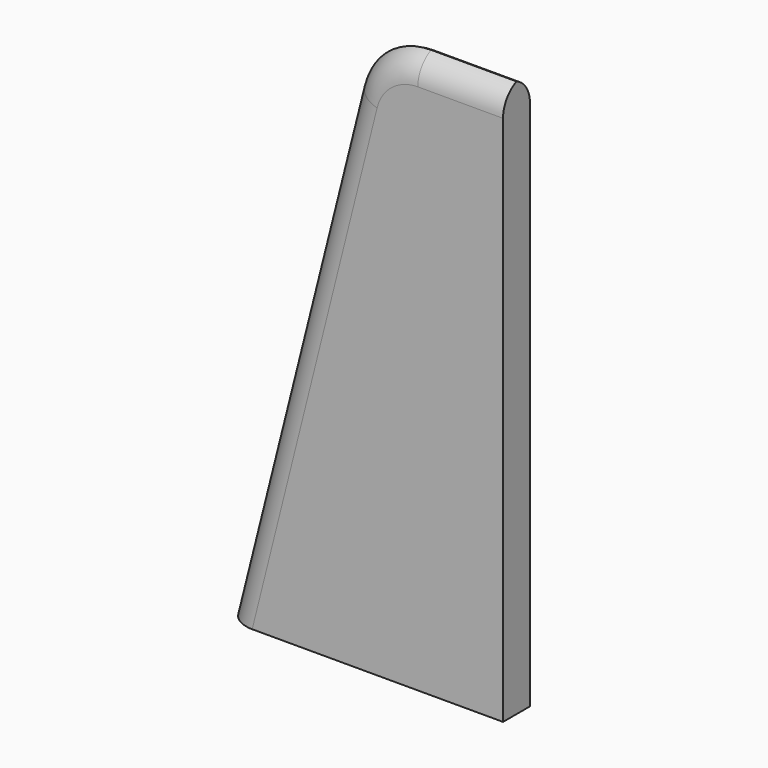
from build123d import *

# Parameters (mm, degrees)
F1_DEPTH    = 3.048
F2_T1_DEPTH = 53.7555112647
F2_T3_DEPTH = 14.0920698193
F2_T6_ANGLE = 75.9637565321
F2_T8_ANGLE = 75.9637565321


# Not quite as in the source:
# - a fillet or chamfer that OpenCascade refuses, or shapes differently, is made with other operations: its cross-section is extruded or revolved along the edge and cut away or added


with BuildPart() as f1:
    # F0 (on Front) → F1 (new body)
    with BuildSketch(Plane.XZ):
        with BuildLine():
            Line((25.4, 50.8), (17.6579301807, 50.8))
            ThreePointArc((17.6579301807, 50.8), (13.750062651, 49.4551045314), (11.4975253047, 45.990101219))
            Line((11.4975253047, 45.990101219), (0, 0))
            Line((0, 0), (25.4, 0))
            Line((25.4, 0), (25.4, 50.8))
        make_face()
    extrude(amount=F1_DEPTH)

    # F2: fillet of radius 2.54 on 2 edges, made by hand

    # F2_s2 → F2_t1 (cut)
    with BuildSketch(Plane(origin=(11.4975253047, 0, 45.990101219), x_dir=(0, 1, 0), z_dir=(-0.242535625, 0, -0.9701425001))):
        with BuildLine():
            ThreePointArc((-0.508, 0), (-2.3040512242, 0.7439487758), (-3.048, 2.54))
            Line((-3.048, 2.54), (-3.048, 0))
            Line((-3.048, 0), (-0.508, 0))
        make_face()
        with BuildLine():
            ThreePointArc((-2.54, 0), (-0.7439487758, 0.7439487758), (0, 2.54))
            Line((0, 2.54), (0, 0))
            Line((0, 0), (-2.54, 0))
        make_face()
    extrude(amount=F2_T1_DEPTH, mode=Mode.SUBTRACT)

    # F2_s4 → F2_t3 (cut)
    with BuildSketch(Plane.YZ.offset(17.6579301807)):
        with BuildLine():
            ThreePointArc((-2.54, 50.8), (-0.7439487758, 50.0560512242), (0, 48.26))
            Line((0, 48.26), (0, 50.8))
            Line((0, 50.8), (-2.54, 50.8))
        make_face()
        with BuildLine():
            ThreePointArc((-0.508, 50.8), (-2.3040512242, 50.0560512242), (-3.048, 48.26))
            Line((-3.048, 48.26), (-3.048, 50.8))
            Line((-3.048, 50.8), (-0.508, 50.8))
        make_face()
    extrude(amount=F2_T3_DEPTH, mode=Mode.SUBTRACT)

    # F2_s5 → F2_t6 (revolve, cut)
    with BuildSketch(Plane.YZ.offset(17.6579301807)):
        with BuildLine():
            ThreePointArc((-2.54, 50.8), (-0.7439487758, 50.0560512242), (0, 48.26))
            Line((0, 48.26), (0, 50.8))
            Line((0, 50.8), (-2.54, 50.8))
        make_face()
    revolve(axis=Axis((17.6579301807, 0, 44.45), (0, -1, 0)), revolution_arc=F2_T6_ANGLE, mode=Mode.SUBTRACT)

    # F2_s7 → F2_t8 (revolve, cut)
    with BuildSketch(Plane.YZ.offset(17.6579301807)):
        with BuildLine():
            ThreePointArc((-0.508, 50.8), (-2.3040512242, 50.0560512242), (-3.048, 48.26))
            Line((-3.048, 48.26), (-3.048, 50.8))
            Line((-3.048, 50.8), (-0.508, 50.8))
        make_face()
    revolve(axis=Axis((17.6579301807, -3.048, 44.45), (0, -1, 0)), revolution_arc=F2_T8_ANGLE, mode=Mode.SUBTRACT)


solid = f1.part
